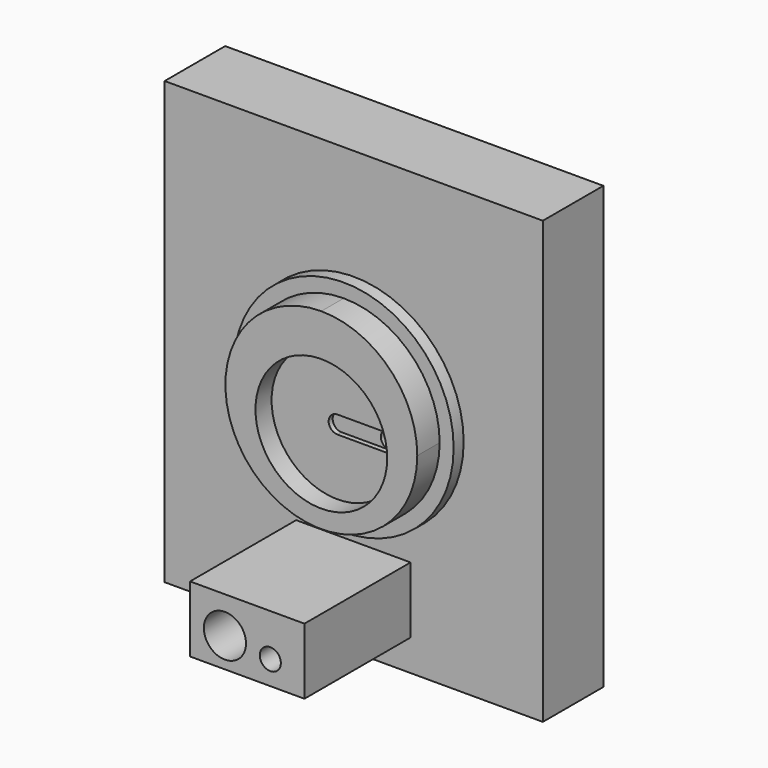
from build123d import *

# Parameters (mm, degrees)
F1_DEPTH  = 4.08178
F0_R      = 11.0744
F2_DEPTH  = 1.26238
F3_R      = 6.63575
F4_DEPTH  = 2.032
F6_DEPTH  = 0.508
F0_W      = 38.1
F0_H      = 44.45
F7_DEPTH  = 7.62
F9_DEPTH  = 27.94
F11_W     = 11.5240756422
F11_H     = 6.661596708
F11_R     = 2.1209
F11_R_2   = 1.0630985687
F12_DEPTH = 13.3604


# Not quite as in the source:
# - ends of sketch curves that miss each other by under 0.0002 mm in the source are joined


with BuildPart() as f1:
    # F0 (on Front) → F1 (new body)
    with BuildSketch(Plane.XZ):
        with BuildLine():
            ThreePointArc((0, 9.6647), (-6.8339749081, -6.8339749081), (9.6647, 0))
            ThreePointArc((9.6647, 0), (6.8339749081, 6.8339749081), (0, 9.6647))
        make_face()
        with BuildLine():
            ThreePointArc((6.63575, -1.21285), (-4.6921838233, -5.9050338233), (0, 5.4229))
            ThreePointArc((0, 5.4229), (4.6921838233, 3.4793338233), (6.63575, -1.21285))
        make_face(mode=Mode.SUBTRACT)
        with BuildLine():
            ThreePointArc((6.63575, -1.21285), (4.6921838233, 3.4793338233), (0, 5.4229))
            ThreePointArc((0, 5.4229), (-4.6921838233, -5.9050338233), (6.63575, -1.21285))
        make_face()
    extrude(amount=F1_DEPTH)

    # F0 (on Front) → F2 (join)
    with BuildSketch(Plane.XZ):
        Circle(F0_R)
        with BuildLine():
            ThreePointArc((0, 9.6647), (6.8339749081, 6.8339749081), (9.6647, 0))
            ThreePointArc((9.6647, 0), (-6.8339749081, -6.8339749081), (0, 9.6647))
        make_face(mode=Mode.SUBTRACT)
    extrude(amount=F2_DEPTH)

    # F3 (on face) → F4 (cut)
    with BuildSketch(Plane.XZ.offset(4.08178)):
        with Locations((0, -1.21285)):
            Circle(F3_R)
    extrude(amount=-F4_DEPTH, mode=Mode.SUBTRACT)

    # F5 (on face) → F6 (cut)
    with BuildSketch(Plane.XZ.offset(2.04978)):
        with BuildLine():
            ThreePointArc((4.8492713831, -0.32385), (4.2206534547, -0.5842320715), (3.9602713831, -1.21285))
            ThreePointArc((3.9602713831, -1.21285), (4.1982717908, -1.818259391), (4.7848395063, -2.0995120175))
            Line((4.7848395063, -2.0995120175), (4.9145697552, -2.0994486254))
            ThreePointArc((4.9145697552, -2.0994486254), (5.5005667281, -1.817941211), (5.7382713831, -1.21285))
            ThreePointArc((5.7382713831, -1.21285), (5.4778893116, -0.5842320715), (4.8492713831, -0.32385))
        make_face()
        with BuildLine():
            ThreePointArc((0, -0.32385), (0.6286179285, -0.5842320715), (0.889, -1.21285))
            Line((0.889, -1.21285), (3.9602713831, -1.21285))
            ThreePointArc((3.9602713831, -1.21285), (4.2206534547, -0.5842320715), (4.8492713831, -0.32385))
            Line((4.8492713831, -0.32385), (0, -0.32385))
        make_face()
        with BuildLine():
            Line((3.9602713831, -1.21285), (0.889, -1.21285))
            ThreePointArc((0.889, -1.21285), (0.6286179285, -0.5842320715), (0, -0.32385))
            ThreePointArc((0, -0.32385), (-0.889, -1.21285), (0, -2.10185))
            Line((0, -2.10185), (4.7848395063, -2.0995120175))
            ThreePointArc((4.7848395063, -2.0995120175), (4.1982717908, -1.818259391), (3.9602713831, -1.21285))
        make_face()
    extrude(amount=-F6_DEPTH, mode=Mode.SUBTRACT)

    # F8 (on face) → F9 (cut)
    with BuildSketch(Plane.XZ.offset(1.54178)):
        with BuildLine():
            Line((4.7848395063, -2.0995120175), (4.9145697552, -2.0994486254))
            ThreePointArc((4.9145697552, -2.0994486254), (5.5005667281, -1.817941211), (5.7382713831, -1.21285))
            ThreePointArc((5.7382713831, -1.21285), (5.4778893116, -0.5842320715), (4.8492713831, -0.32385))
            ThreePointArc((4.8492713831, -0.32385), (3.960856071, -1.1806128595), (4.7848395063, -2.0995120175))
        make_face()
    extrude(amount=-F9_DEPTH, mode=Mode.SUBTRACT)


with BuildPart() as f7:
    # F0 (on Front) → F7 (new body)
    with BuildSketch(Plane.XZ):
        Rectangle(F0_W, F0_H)
        Circle(F0_R, mode=Mode.SUBTRACT)
    extrude(amount=-F7_DEPTH)

    # F11 (on face) → F12 (join)
    with BuildSketch(Plane.XZ):
        with Locations((-0.0403500162, -15.7439657487)):
            Rectangle(F11_W, F11_H)
        with Locations((-2.289429307, -16.0906407982)):
            Circle(F11_R, mode=Mode.SUBTRACT)
        with Locations((2.2835119162, -16.6806168854)):
            Circle(F11_R_2, mode=Mode.SUBTRACT)
    extrude(amount=F12_DEPTH)


solid = Compound([f1.part, f7.part])
